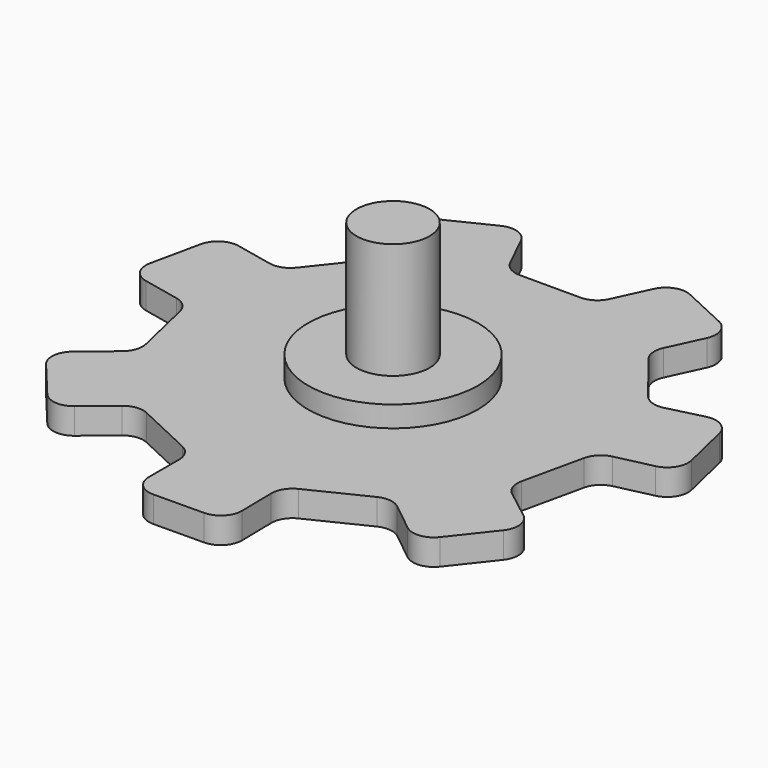
from build123d import *

# Parameters (mm, degrees)
F1_DEPTH = 2.54
F2_SCALE = 1.12
F3_R     = 1.27
F4_R     = 2.2098
F5_DEPTH = 7.0104
F6_ANGLE = 180
F7_DEPTH = 1.27
F8_R     = 5.1308
F8_R_2   = 2.2098
F9_DEPTH = 1.27


with BuildPart() as f1:
    # F0 (on Top) → F1 (new body)
    with BuildSketch(Plane.XY):
        Polygon((2.6097216178, 14.5627437159), (-2.4016266689, 14.6046923473), (-2.4016266689, 10.7069099322), (-6.7973635159, 8.6464090273), (-9.7507489845, 11.1018400639), (-12.9371215583, 7.269280193), (-9.9187448393, 4.759815731), (-10.987800546, 0.1461525389), (-14.7898914292, -0.6685812259), (-13.7329729143, -5.6008676039), (-9.9187448393, -4.7835330123), (-6.9650523365, -8.5103949532), (-8.662414737, -11.9730141014), (-4.136644538, -14.1915290003), (-2.4166579341, -10.6827564792), (2.3025460541, -10.6827564792), (3.9659612812, -14.2644541338), (8.5153820935, -12.1516080526), (6.8819414162, -8.6344521752), (9.8897544667, -4.8440932296), (13.6239528656, -5.7776425965), (14.7675592452, -0.8934023208), (10.9942825511, -0.0382388607), (9.9505092949, 4.6697063372), (13.008704409, 7.0334360935), (9.9016642198, 10.9836040065), (6.8838195875, 8.5752755404), (2.5481330231, 10.6975259259), align=None)
    extrude(amount=F1_DEPTH)


with BuildPart() as f1_1:
    # F2: moved
    add(f1.part.scale(F2_SCALE))

    # F3
    f3_edges = [f1_1.edges().sort_by_distance(p)[0] for p in [
        (-16.564678, -0.748811, 1.4224),
        (-12.306337, 0.163691, 1.4224),
        (-14.489576, 8.141594, 1.4224),
        (-10.920839, 12.434061, 1.4224),
        (-7.613047, 9.683978, 1.4224),
        (-2.689822, 11.991739, 1.4224),
        (-2.689822, 16.357255, 1.4224),
        (2.922888, 16.310273, 1.4224),
        (2.853909, 11.981229, 1.4224),
        (7.709878, 9.604309, 1.4224),
        (11.089864, 12.301636, 1.4224),
        (14.569749, 7.877448, 1.4224),
        (11.14457, 5.230071, 1.4224),
        (12.313596, -0.042828, 1.4224),
        (16.539666, -1.000611, 1.4224),
        (15.258827, -6.47096, 1.4224),
        (11.076525, -5.425384, 1.4224),
        (7.707774, -9.670586, 1.4224),
        (9.537228, -13.609801, 1.4224),
        (4.441877, -15.976189, 1.4224),
        (2.578852, -11.964687, 1.4224),
        (-2.706657, -11.964687, 1.4224),
        (-4.633042, -15.894512, 1.4224),
        (-9.701905, -13.409776, 1.4224),
        (-7.800859, -9.531642, 1.4224),
        (-11.108994, -5.357557, 1.4224),
        (-15.38093, -6.272972, 1.4224),
        (-11.108994, 5.330994, 1.4224),
    ]]
    fillet(f3_edges, radius=F3_R)

    # F4 (on face) → F5 (join)
    with BuildSketch(Plane.XY):
        Circle(F4_R)
    extrude(amount=-F5_DEPTH)


with BuildPart() as f1_2:
    # F6: moved
    add(f1_1.part.rotate(Axis((-0.0732200051, -11.9646872567, 0), (1, 0, 0)), F6_ANGLE))

    # F7 (cut): a face of the model
    f7_faces = [f1_2.faces().sort_by_distance(p)[0] for p in [
        (5.0824398182, -34.3118398385, 0),
    ]]
    extrude(f7_faces, amount=-F7_DEPTH, mode=Mode.SUBTRACT)

    # F8 (on face) → F9 (join)
    with BuildSketch(Plane.XY.offset(-1.27)):
        with Locations((0, -23.9293745135)):
            Circle(F8_R)
        with Locations((0, -23.9293745135)):
            Circle(F8_R_2, mode=Mode.SUBTRACT)
    extrude(amount=F9_DEPTH)


solid = f1_2.part
